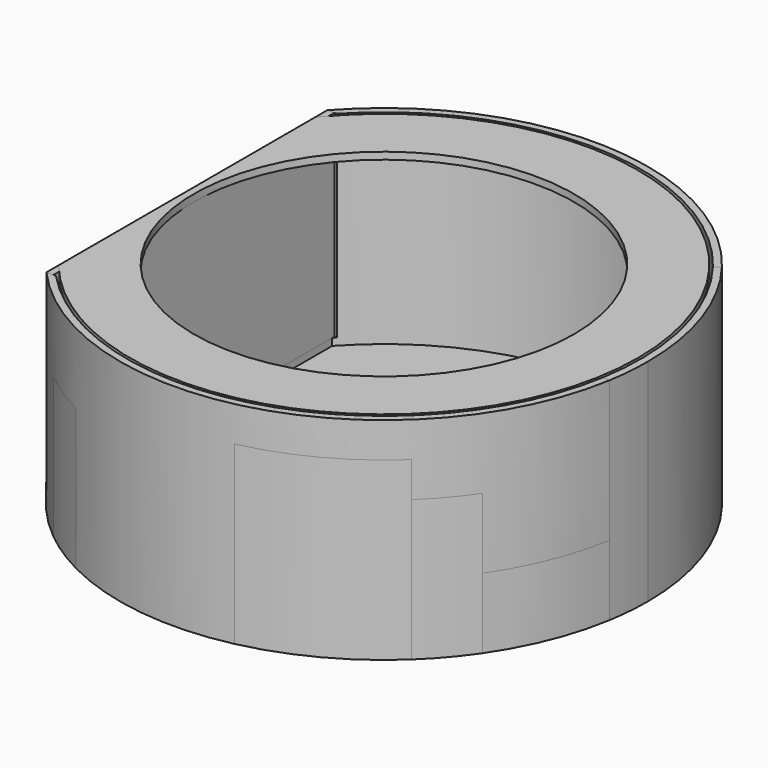
from build123d import *

# Parameters (mm, degrees)
F0_R        = 37.5
F1_DEPTH    = 30
F3_DEPTH    = 28
F8_T        = 1
F8_T3_DEPTH = 51.8898787331
F9_DEPTH    = 20
F10_DEPTH   = 20
F11_DEPTH   = 25
F12_DEPTH   = 25
F13_DEPTH   = 10
F14_DEPTH   = 10
F15_DEPTH   = 30
F16_DEPTH   = 30
F17_DEPTH   = 20
F18_DEPTH   = 20
F19_W       = 49.8898787331
F19_H       = 28
F20_DEPTH   = 1.3551748111
F21_DEPTH   = 1
F4_R        = 27
F22_DEPTH   = 1


# Not quite as in the source:
# - a shell that OpenCascade refuses in one call is made with other operations: the cavity is built on its own and cut out


with BuildPart() as f1:
    # F0 (on Top) → F1 (new body)
    with BuildSketch(Plane.XY):
        Circle(F0_R)
    extrude(amount=-F1_DEPTH)

    # F2 (on face) → F3 (cut)
    with BuildSketch(Plane.XY):
        with BuildLine():
            Line((-28, -24.9449393665), (-28, 24.9449393665))
            ThreePointArc((-28, 24.9449393665), (-37.5, 0), (-28, -24.9449393665))
        make_face()
    extrude(amount=-F3_DEPTH, mode=Mode.SUBTRACT)

    # F8: shell of thickness 1, made by hand


with BuildPart() as f8_core1:
    # F8_t2: copy of F1
    add(f1.part)

    # the walls: a layer under each face that stays
    f8_faces = [f8_core1.faces().sort_by_distance(p)[0] for p in [
        (18.75, 32.4759526419, -25),
        (-28, 0, -14),
        (-32.75, 0, -28),
        (0, 0, -30),
    ]]
    thicken(f8_faces, amount=-F8_T, mode=Mode.SUBTRACT)

    # F8_s4 → F8_t3 (cut)
    with BuildSketch(Plane.XZ.offset(-25.9449393665)):
        Polygon((-28.01, -27.99), (-27, -28), (-27, -29), (-28, -29), align=None)
    extrude(amount=F8_T3_DEPTH, mode=Mode.SUBTRACT)


with BuildPart() as f1_1:
    add(f1.part)

    # what is left inside the walls is the cavity
    f8_cavity = [f8_core1.part.solids().sort_by_distance(p)[0] for p in [
        (36.49, 0, -19.333333),
    ]]
    add(f8_cavity, mode=Mode.SUBTRACT)

    # F6 (on face) → F9 (cut)
    with BuildSketch(Plane(origin=(0, 0, -30), x_dir=(1, 0, 0), z_dir=(0, 0, -1))):
        with BuildLine():
            ThreePointArc((-16.953998922, 33.4486460197), (-20.4251291644, 31.4493894793), (-23.6632020109, 29.0912851313))
            Line((-23.6632020109, 29.0912851313), (-23.0321832906, 28.3155175278))
            ThreePointArc((-23.0321832906, 28.3155175278), (-19.8804590533, 30.6107390931), (-16.501892284, 32.5566821259))
            Line((-16.501892284, 32.5566821259), (-16.953998922, 33.4486460197))
        make_face()
    extrude(amount=-F9_DEPTH, mode=Mode.SUBTRACT)

    # F7 (on face) → F11 (cut)
    with BuildSketch(Plane(origin=(0, 0, -30), x_dir=(1, 0, 0), z_dir=(0, 0, -1))):
        with BuildLine():
            ThreePointArc((25.7285399775, 27.2817197153), (17.5217539189, 33.1547604365), (8.046001078, 36.6266551387))
            Line((8.046001078, 36.6266551387), (6.8659209199, 31.2547457184))
            ThreePointArc((6.8659209199, 31.2547457184), (14.9518966775, 28.2920622392), (21.9550207808, 23.2804008237))
            Line((21.9550207808, 23.2804008237), (25.0424455781, 26.5542071896))
            Line((25.0424455781, 26.5542071896), (25.7285399775, 27.2817197153))
        make_face()
    extrude(amount=-F11_DEPTH, mode=Mode.SUBTRACT)

    # F7 (on face) → F13 (cut)
    with BuildSketch(Plane(origin=(0, 0, -30), x_dir=(1, 0, 0), z_dir=(0, 0, -1))):
        with BuildLine():
            ThreePointArc((36.9833338658, 6.2034680763), (34.7750507424, 14.0337395539), (30.9299683404, 21.2034680763))
            Line((30.9299683404, 21.2034680763), (30.1051691846, 20.638042261))
            Line((30.1051691846, 20.638042261), (26.3935729838, 18.0936260918))
            ThreePointArc((26.3935729838, 18.0936260918), (29.6747099668, 11.9754577526), (31.5591115654, 5.2936260918))
            Line((31.5591115654, 5.2936260918), (35.9971116293, 6.038042261))
            Line((35.9971116293, 6.038042261), (36.9833338658, 6.2034680763))
        make_face()
    extrude(amount=-F13_DEPTH, mode=Mode.SUBTRACT)

    # F7 (on face) → F15 (cut)
    with BuildSketch(Plane(origin=(0, 0, -30), x_dir=(1, 0, 0), z_dir=(0, 0, -1))):
        with BuildLine():
            Line((28.9052016216, -22.2876494771), (29.6971249537, -22.8982700107))
            ThreePointArc((29.6971249537, -22.8982700107), (35.49571936, -12.0956152021), (37.5, 0))
            ThreePointArc((37.5, 0), (37.3706102437, 3.1124732958), (36.9833338658, 6.2034680763))
            Line((36.9833338658, 6.2034680763), (35.9971116293, 6.038042261))
            ThreePointArc((35.9971116293, 6.038042261), (35.4071146726, -8.8648875097), (28.9052016216, -22.2876494771))
        make_face()
    extrude(amount=-F15_DEPTH, mode=Mode.SUBTRACT)

    # F7 (on face) → F17 (cut)
    with BuildSketch(Plane(origin=(0, 0, -30), x_dir=(1, 0, 0), z_dir=(0, 0, -1))):
        with BuildLine():
            ThreePointArc((30.9299683404, 21.2034680763), (28.4918045576, 24.3816954507), (25.7285399775, 27.2817197153))
            Line((25.7285399775, 27.2817197153), (25.0424455781, 26.5542071896))
            ThreePointArc((25.0424455781, 26.5542071896), (27.7320231027, 23.7315169054), (30.1051691846, 20.638042261))
            Line((30.1051691846, 20.638042261), (30.9299683404, 21.2034680763))
        make_face()
    extrude(amount=-F17_DEPTH, mode=Mode.SUBTRACT)

    # F19 (on face) → F20 (cut, through all)
    with BuildSketch(Plane(origin=(-28, 0, 0), x_dir=(0, -1, 0), z_dir=(-1, 0, 0))):
        with Locations((0, -14)):
            Rectangle(F19_W, F19_H)
    extrude(amount=-F20_DEPTH, mode=Mode.SUBTRACT)


with BuildPart() as f10:
    # F6 (on face) → F10 (new body)
    with BuildSketch(Plane(origin=(0, 0, -30), x_dir=(1, 0, 0), z_dir=(0, 0, -1))):
        with BuildLine():
            ThreePointArc((-16.953998922, 33.4486460197), (-20.4251291644, 31.4493894793), (-23.6632020109, 29.0912851313))
            Line((-23.6632020109, 29.0912851313), (-23.0321832906, 28.3155175278))
            ThreePointArc((-23.0321832906, 28.3155175278), (-19.8804590533, 30.6107390931), (-16.501892284, 32.5566821259))
            Line((-16.501892284, 32.5566821259), (-16.953998922, 33.4486460197))
        make_face()
    extrude(amount=-F10_DEPTH)


with BuildPart() as f12:
    # F7 (on face) → F12 (new body)
    with BuildSketch(Plane(origin=(0, 0, -30), x_dir=(1, 0, 0), z_dir=(0, 0, -1))):
        with BuildLine():
            ThreePointArc((25.7285399775, 27.2817197153), (17.5217539189, 33.1547604365), (8.046001078, 36.6266551387))
            Line((8.046001078, 36.6266551387), (6.8659209199, 31.2547457184))
            ThreePointArc((6.8659209199, 31.2547457184), (14.9518966775, 28.2920622392), (21.9550207808, 23.2804008237))
            Line((21.9550207808, 23.2804008237), (25.0424455781, 26.5542071896))
            Line((25.0424455781, 26.5542071896), (25.7285399775, 27.2817197153))
        make_face()
    extrude(amount=-F12_DEPTH)


with BuildPart() as f14:
    # F7 (on face) → F14 (new body)
    with BuildSketch(Plane(origin=(0, 0, -30), x_dir=(1, 0, 0), z_dir=(0, 0, -1))):
        with BuildLine():
            ThreePointArc((36.9833338658, 6.2034680763), (34.7750507424, 14.0337395539), (30.9299683404, 21.2034680763))
            Line((30.9299683404, 21.2034680763), (30.1051691846, 20.638042261))
            Line((30.1051691846, 20.638042261), (26.3935729838, 18.0936260918))
            ThreePointArc((26.3935729838, 18.0936260918), (29.6747099668, 11.9754577526), (31.5591115654, 5.2936260918))
            Line((31.5591115654, 5.2936260918), (35.9971116293, 6.038042261))
            Line((35.9971116293, 6.038042261), (36.9833338658, 6.2034680763))
        make_face()
    extrude(amount=-F14_DEPTH)


with BuildPart() as f16:
    # F7 (on face) → F16 (new body)
    with BuildSketch(Plane(origin=(0, 0, -30), x_dir=(1, 0, 0), z_dir=(0, 0, -1))):
        with BuildLine():
            Line((28.9052016216, -22.2876494771), (29.6971249537, -22.8982700107))
            ThreePointArc((29.6971249537, -22.8982700107), (35.49571936, -12.0956152021), (37.5, 0))
            ThreePointArc((37.5, 0), (37.3706102437, 3.1124732958), (36.9833338658, 6.2034680763))
            Line((36.9833338658, 6.2034680763), (35.9971116293, 6.038042261))
            ThreePointArc((35.9971116293, 6.038042261), (35.4071146726, -8.8648875097), (28.9052016216, -22.2876494771))
        make_face()
    extrude(amount=-F16_DEPTH)


with BuildPart() as f18:
    # F7 (on face) → F18 (new body)
    with BuildSketch(Plane(origin=(0, 0, -30), x_dir=(1, 0, 0), z_dir=(0, 0, -1))):
        with BuildLine():
            ThreePointArc((30.9299683404, 21.2034680763), (28.4918045576, 24.3816954507), (25.7285399775, 27.2817197153))
            Line((25.7285399775, 27.2817197153), (25.0424455781, 26.5542071896))
            ThreePointArc((25.0424455781, 26.5542071896), (27.7320231027, 23.7315169054), (30.1051691846, 20.638042261))
            Line((30.1051691846, 20.638042261), (30.9299683404, 21.2034680763))
        make_face()
    extrude(amount=-F18_DEPTH)


with BuildPart() as f21:
    # F19 (on face) → F21 (new body)
    with BuildSketch(Plane(origin=(-28, 0, 0), x_dir=(0, -1, 0), z_dir=(-1, 0, 0))):
        with Locations((0, -14)):
            Rectangle(F19_W, F19_H)
    extrude(amount=-F21_DEPTH)


with BuildPart() as f22:
    # F4 (on face) → F22 (new body)
    with BuildSketch(Plane.XY):
        with BuildLine():
            ThreePointArc((-28, -22.7861800221), (36.1, 0), (-28, 22.7861800221))
            Line((-28, 22.7861800221), (-28, -22.7861800221))
        make_face()
        Circle(F4_R, mode=Mode.SUBTRACT)
    extrude(amount=-F22_DEPTH)


solid = Compound([f1_1.part, f10.part, f12.part, f14.part, f16.part, f18.part, f21.part, f22.part])
